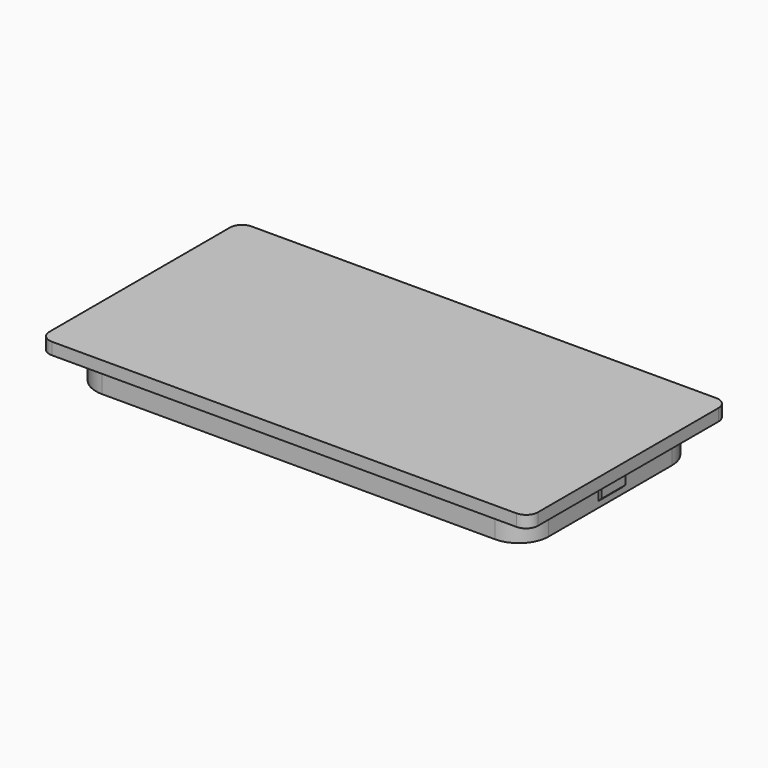
from build123d import *

# Parameters (mm, degrees)
F0_W      = 75.8
F0_H      = 35.8
F0_W_2    = 71.8000013767
F0_H_2    = 31.8
F1_DEPTH  = 5
F2_W      = 3
F2_H      = 3
F3_DEPTH  = 2
F4_R      = 5
F5_R      = 10
F6_R      = 2
F7_W      = 5
F7_H      = 2
F8_DEPTH  = 0.5
F9_W      = 5
F9_H      = 2
F10_DEPTH = 0.5
F11_SIZE  = 0.49999


# Not quite as in the source:
# - a fillet or chamfer is up to 0.001 mm smaller than in the source, because OpenCascade refuses the exact size


with BuildPart() as f1:
    # F0 (on Top) → F1 (new body)
    with BuildSketch(Plane.XY):
        with Locations((-3.8991395473, 2.3895057946)):
            Rectangle(F0_W, F0_H)
        with Locations((-3.8991395473, 2.3895057946)):
            Rectangle(F0_W_2, F0_H_2, mode=Mode.SUBTRACT)
    extrude(amount=F1_DEPTH)

    # F2 (on face) → F3 (join)
    with BuildSketch(Plane.XY.offset(5)):
        Polygon((37.0008604527, 23.2895057946), (-44.7991395473, 23.2895057946), (-44.7991395473, -18.5104942054), (34.0008604527, -18.5104942054), (34.0008604527, -15.5104942054), (37.0008604527, -15.5104942054), align=None)
        with Locations((35.5008604527, -17.0104942054)):
            Rectangle(F2_W, F2_H)
    extrude(amount=F3_DEPTH)

    # F4
    f4_edges = [f1.edges().sort_by_distance(p)[0] for p in [
        (34.00086, 20.289506, 2.5),
        (34.00086, -15.510494, 2.5),
        (-41.79914, -15.510494, 2.5),
        (-41.79914, 20.289506, 2.5),
    ]]
    fillet(f4_edges, radius=F4_R)

    # F5
    f5_edges = [f1.edges().sort_by_distance(p)[0] for p in [
        (32.000861, -13.510494, 2.5),
        (32.000861, 18.289506, 2.5),
        (-39.79914, 18.289506, 2.5),
        (-39.79914, -13.510494, 2.5),
    ]]
    fillet(f5_edges, radius=F5_R)

    # F6
    f6_edges = [f1.edges().sort_by_distance(p)[0] for p in [
        (37.00086, -18.510494, 6),
        (37.00086, 23.289506, 6),
        (-44.79914, 23.289506, 6),
        (-44.79914, -18.510494, 6),
    ]]
    fillet(f6_edges, radius=F6_R)

    # F7 (on face) → F8 (join)
    with BuildSketch(Plane(origin=(-41.7991395473, 0, 0), x_dir=(0, -1, 0), z_dir=(-1, 0, 0))):
        with Locations((-2.3895057946, 2)):
            Rectangle(F7_W, F7_H)
    extrude(amount=F8_DEPTH)

    # F9 (on face) → F10 (join)
    with BuildSketch(Plane.YZ.offset(34.0008604527)):
        with Locations((2.3895057946, 2)):
            Rectangle(F9_W, F9_H)
    extrude(amount=F10_DEPTH)

    # F11 (size 0.5 in the source; OpenCascade refuses exactly that, so slightly less here)
    f11_edges = [f1.edges().sort_by_distance(p)[0] for p in [
        (34.50086, 2.389506, 1),
        (-42.29914, 2.389506, 1),
    ]]
    chamfer(f11_edges, length=F11_SIZE)


solid = f1.part
